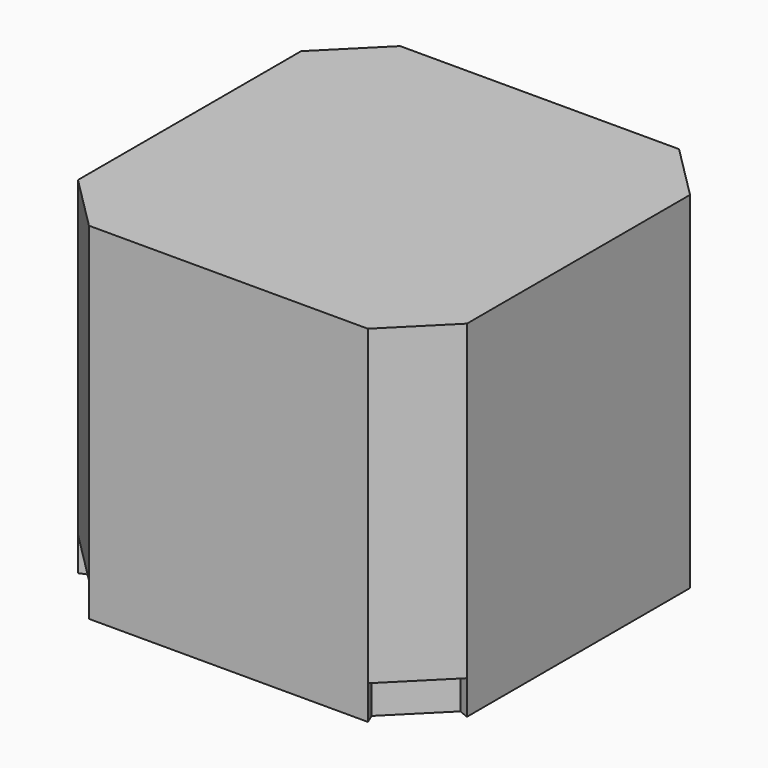
from build123d import *

# Parameters (mm, degrees)
F1_DEPTH = 89
F3_DEPTH = 8.75
F4_T     = -2.5


# Not quite as in the source:
# - a shell that OpenCascade refuses in one call is made with other operations: the cavity is built on its own and cut out


with BuildPart() as f1:
    # F0 (on Top) → F1 (new body)
    with BuildSketch(Plane.XY):
        Polygon((50, 35.8578643763), (35.8578643763, 50), (-35.8578643763, 50), (-50, 35.8578643763), (-50, -35.8578643763), (-35.8578643763, -50), (35.8578643763, -50), (50, -35.8578643763), align=None)
    extrude(amount=-F1_DEPTH)

    # F2 (on face) → F3 (cut)
    with BuildSketch(Plane(origin=(0, 0, -89), x_dir=(1, 0, 0), z_dir=(0, 0, -1))):
        Polygon((-50, 35.8578643763), (-47.5, 34.8223305494), (-34.8223305494, 47.5), (-35.8578643763, 50), align=None)
        Polygon((-47.5, -34.8223304703), (-50, -35.8578643763), (-35.8578643763, -50), (-34.8223304703, -47.5), align=None)
        Polygon((50, 35.8578643763), (35.8578643763, 50), (34.8223305494, 47.5), (47.5, 34.8223305494), align=None)
        Polygon((34.8223305494, -47.5), (35.8578643763, -50), (50, -35.8578643763), (47.5, -34.8223305494), align=None)
    extrude(amount=-F3_DEPTH, mode=Mode.SUBTRACT)

    # F4: a shell. OpenCascade refuses it in one call, so the cavity is built on its own and cut out:
    # the body offset inwards by the wall thickness, plus a prism from it out through each open face.
    f4_core = offset(f1.part, amount=F4_T, kind=Kind.INTERSECTION, mode=Mode.PRIVATE)
    f4_exits = [f4_core.faces().sort_by_distance(p)[0] for p in [
        (0, 0, -86.5),
    ]]
    add(f4_core, mode=Mode.SUBTRACT)
    extrude(f4_exits, amount=-F4_T, mode=Mode.SUBTRACT)


solid = f1.part
